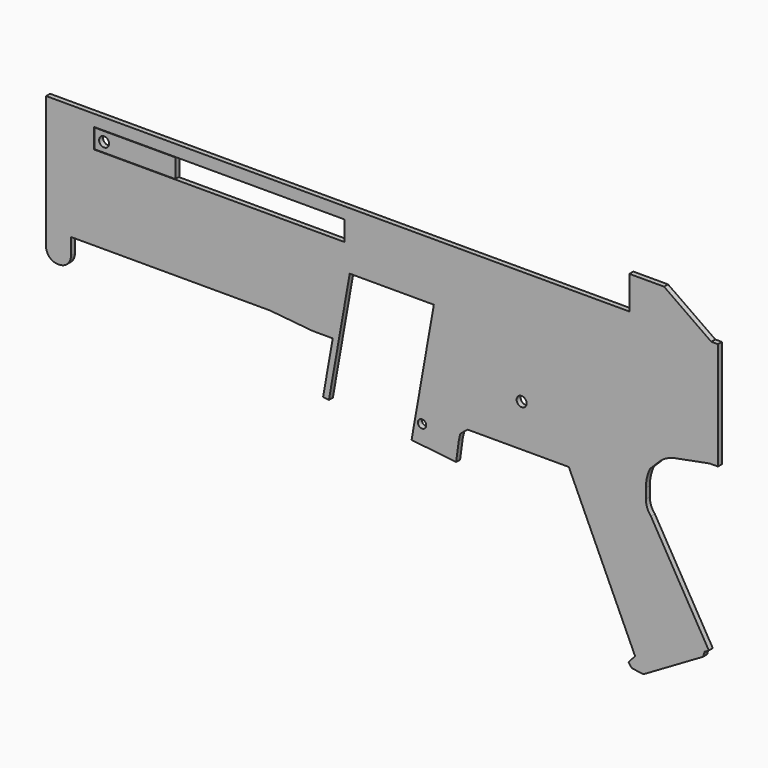
from build123d import *

# Parameters (mm, degrees)
F0_R     = 2.5
F0_W     = 151
F0_H     = 12
F0_R_2   = 3
F1_DEPTH = 3
F0_W_2   = 48.75
F0_H_2   = 11.5


# Not quite as in the source:
# - a feature names something its author has since deleted; it is built from what else it names


with BuildPart() as f1:
    # F0 (on Front) → F1 (new body)
    with BuildSketch(Plane.XZ):
        with BuildLine():
            Line((48.4706909373, -65), (53.4706909373, -65))
            Line((53.4706909373, -65), (53.4706909373, 0))
            Line((53.4706909373, 0), (49.4706909373, 0))
            Line((49.4706909373, 0), (20.9706909373, 19.9999785245))
            Line((20.9706909373, 19.9999785245), (-0.0293090627, 19.9999785245))
            Line((-0.0293090627, 19.9999785245), (0, 0))
            Line((0, 0), (-352, 0))
            Line((-352, 0), (-352, -39))
            Line((-352, -39), (-352, -55.5))
            Line((-352, -55.5), (-352, -80))
            ThreePointArc((-352, -80), (-349.9497474683, -84.9497474683), (-345, -87))
            Line((-345, -87), (-344, -87))
            ThreePointArc((-344, -87), (-339.0502525317, -84.9497474683), (-337, -80))
            Line((-337, -80), (-337, -70))
            Line((-337, -70), (-217, -70))
            Line((-217, -70), (-191, -72.5))
            Line((-191, -72.5), (-179, -72.5))
            Line((-179, -72.5), (-184.8187903634, -105.5))
            Line((-184.8187903634, -105.5), (-181.3187903634, -106))
            Line((-181.3187903634, -106), (-172.4142778376, -55.5))
            Line((-172.4142778376, -55.5), (-168.7590112311, -34.7699529486))
            Line((-168.7590112311, -34.7699529486), (-117.9876806368, -34.7699529486))
            Line((-117.9876806368, -34.7699529486), (-118.692445624, -38.7668738074))
            Line((-118.692445624, -38.7668738074), (-121.6429472433, -55.5))
            Line((-121.6429472433, -55.5), (-131.4303426842, -111.007077825))
            Line((-131.4303426842, -111.007077825), (-104.5337054221, -114))
            Line((-104.5337054221, -114), (-103, -102.5))
            Line((-103, -102.5), (-102, -98))
            Line((-102, -98), (-97.5, -94.5))
            Line((-97.5, -94.5), (-36.5, -94.5))
            Line((-36.5, -94.5), (3.4706909373, -182))
            Line((3.4706909373, -182), (-0.5293090627, -186.5))
            Line((-0.5293090627, -186.5), (1.4706909373, -189))
            Line((1.4706909373, -189), (8.4706909373, -190))
            Line((8.4706909373, -190), (44.4706909373, -169))
            Line((44.4706909373, -169), (45.4706909373, -166))
            Line((45.4706909373, -166), (47.9706909373, -164.5))
            Line((47.9706909373, -164.5), (12.9706909373, -104.5))
            ThreePointArc((12.9706909373, -104.5), (10.7453526102, -100.7720018727), (9.9706909373, -96.5))
            Line((9.9706909373, -96.5), (9.9706909373, -90.5))
            ThreePointArc((9.9706909373, -90.5), (10.6035597574, -84.8597429137), (12.4706909373, -79.5))
            Line((12.4706909373, -79.5), (18.4706909373, -73.5))
            ThreePointArc((18.4706909373, -73.5), (22.6588628123, -70.6263437501), (27.4706909373, -69))
            Line((27.4706909373, -69), (48.4706909373, -65))
        make_face()
        with Locations((-125.101, -100.41)):
            Circle(F0_R, mode=Mode.SUBTRACT)
        with Locations((-247.5, -13)):
            Rectangle(F0_W, F0_H, mode=Mode.SUBTRACT)
        with Locations((-65, -69)):
            Circle(F0_R_2, mode=Mode.SUBTRACT)
    extrude(amount=F1_DEPTH)


with BuildPart() as f1b:
    # F0 (on Front) → F1, piece 2 (new body)
    with BuildSketch(Plane.XZ):
        with Locations((-298.375, -13)):
            Rectangle(F0_W_2, F0_H_2)
        with Locations((-317, -13)):
            Circle(F0_R_2, mode=Mode.SUBTRACT)
    extrude(amount=F1_DEPTH)


solid = Compound([f1.part, f1b.part])
